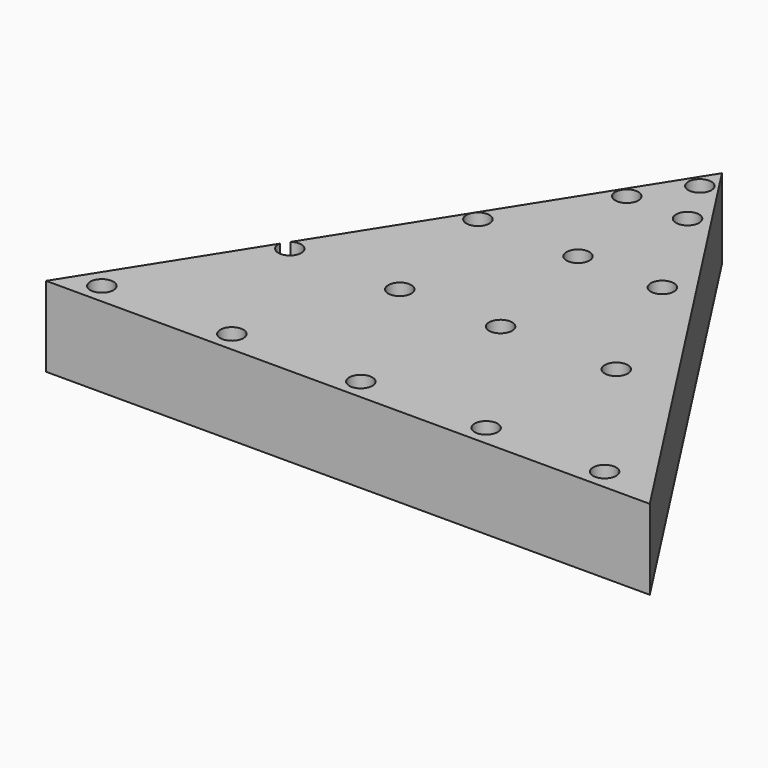
from build123d import *

# Parameters (mm, degrees)
F1_DEPTH = 12.7
F2_R     = 1.8288
F3_DEPTH = 5.08


# Not quite as in the source:
# - the program builds the solid bodies; features that only make, move or delete a surface that nothing else refers to are left out


with BuildPart() as f1:
    # F0 (on Top) → F1 (new body)
    with BuildSketch(Plane.XY):
        Polygon((48.4242066741, -22.2311150283), (0, 52.6062995195), (-47.3236590624, -22.2311150283), align=None)
    extrude(amount=F1_DEPTH)

    # F2 (on face) → F3 (cut)
    with BuildSketch(Plane.XY.offset(12.7)):
        with Locations((-41.0783812404, -18.9761463553)):
            Circle(F2_R)
        with Locations((-20.4600691795, -18.9761463553)):
            Circle(F2_R)
        with Locations((0, -18.9761463553)):
            Circle(F2_R)
        with Locations((19.8642425239, -18.9761463553)):
            Circle(F2_R)
        with Locations((38.6579222977, -18.9761463553)):
            Circle(F2_R)
        with Locations((-29.1365217417, 3.3634696156)):
            Circle(F2_R)
        with Locations((-11.6957994178, 3.3634696156)):
            Circle(F2_R)
        with Locations((4.2915293016, 3.3634696156)):
            Circle(F2_R)
        with Locations((22.6406212896, 3.3634696156)):
            Circle(F2_R)
        with Locations((-15.87430574, 24.0743272007)):
            Circle(F2_R)
        with Locations((0, 24.0743272007)):
            Circle(F2_R)
        with Locations((13.3752385154, 24.0743272007)):
            Circle(F2_R)
        with Locations((-5.3372029215, 40.4250063002)):
            Circle(F2_R)
        with Locations((4.2915293016, 40.4250063002)):
            Circle(F2_R)
        with Locations((0, 48.2369959354)):
            Circle(F2_R)
    extrude(amount=-F3_DEPTH, mode=Mode.SUBTRACT)


solid = f1.part
